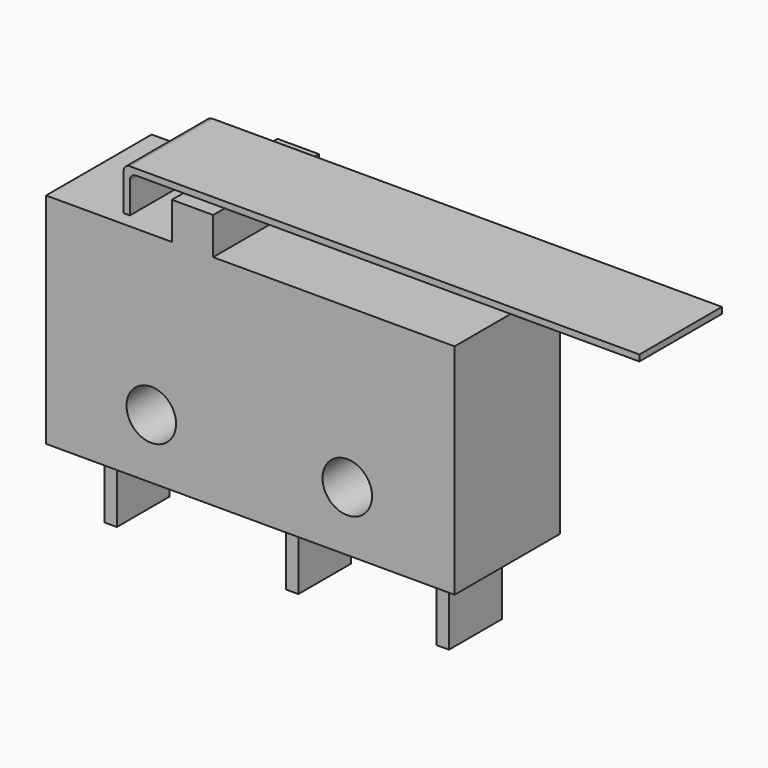
from build123d import *

# Parameters (mm, degrees)
F0_R     = 1.2
F1_DEPTH = 6.4
F2_W     = 0.6
F2_H     = 3.2
F3_DEPTH = 3.5
F4_W     = 25
F4_H     = 5
F5_DEPTH = 0.3
F6_W     = 0.3
F6_H     = 5
F7_DEPTH = 3
F8_R     = 0.3


with BuildPart() as f1:
    # F0 (on Front) → F1 (new body)
    with BuildSketch(Plane.XZ):
        Polygon((0, 10.6), (0, 0), (19.8, 0), (19.8, 10.6), (8.1, 10.6), (8.1, 12.4), (6.1, 12.4), (6.1, 10.6), align=None)
        with Locations((5.1, 2.9)):
            Circle(F0_R, mode=Mode.SUBTRACT)
        with Locations((14.6, 2.9)):
            Circle(F0_R, mode=Mode.SUBTRACT)
    extrude(amount=F1_DEPTH)


with BuildPart() as f3:
    # F2 (on face) → F3 (new body)
    with BuildSketch(Plane(origin=(0, 0, 0), x_dir=(1, 0, 0), z_dir=(0, 0, -1))):
        with Locations((1.85, 3.2)):
            Rectangle(F2_W, F2_H)
    extrude(amount=F3_DEPTH)


with BuildPart() as f3b:
    # F2 (on face) → F3, piece 2 (new body)
    with BuildSketch(Plane(origin=(0, 0, 0), x_dir=(1, 0, 0), z_dir=(0, 0, -1))):
        with Locations((10.65, 3.2)):
            Rectangle(F2_W, F2_H)
    extrude(amount=F3_DEPTH)


with BuildPart() as f3c:
    # F2 (on face) → F3, piece 3 (new body)
    with BuildSketch(Plane(origin=(0, 0, 0), x_dir=(1, 0, 0), z_dir=(0, 0, -1))):
        with Locations((17.95, 3.2)):
            Rectangle(F2_W, F2_H)
    extrude(amount=F3_DEPTH)


with BuildPart() as f5:
    # F4 (on face) → F5 (new body)
    with BuildSketch(Plane.XY.offset(12.4)):
        with Locations((15.7, -3.2)):
            Rectangle(F4_W, F4_H)
    extrude(amount=F5_DEPTH)

    # F6 (on face) → F7 (join)
    with BuildSketch(Plane.XY.offset(12.7)):
        with Locations((3.35, -3.2)):
            Rectangle(F6_W, F6_H)
    extrude(amount=-F7_DEPTH)

    # F8
    f8_edges = [f5.edges().sort_by_distance(p)[0] for p in [
        (3.2, -3.2, 12.7),
        (3.5, -3.2, 12.4),
    ]]
    fillet(f8_edges, radius=F8_R)


solid = Compound([f1.part, f3.part, f3b.part, f3c.part, f5.part])
